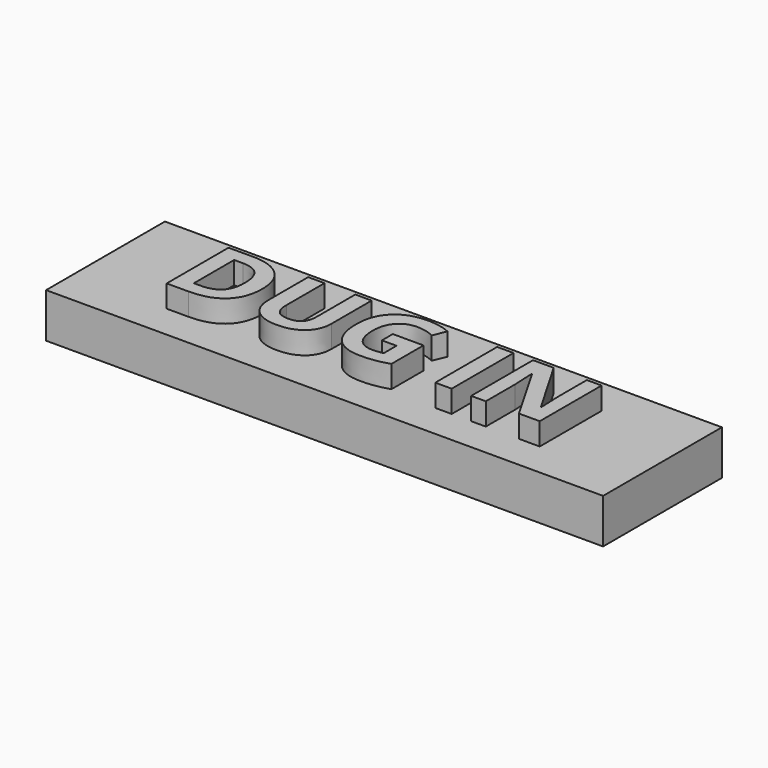
from build123d import *

# Parameters (mm, degrees)
F0_W         = 25
F0_H         = 6.6666666667
F1_DEPTH     = 2
F2_TEXT_SIZE = 4.8611111111
F3_DEPTH     = 1


# Not quite as in the source:
# - Text() gives the source's letters only with a copy of the font that has no kerning and outlines rounded to 1/6400 em; it was checked with that copy


with BuildPart() as f1:
    # F0 (on Top) → F1 (new body)
    with BuildSketch(Plane.XY):
        with Locations((-38.2137671113, 26.4245305329)):
            Rectangle(F0_W, F0_H)
    extrude(amount=F1_DEPTH)

    # F2 (on face) → F3 (join)
    with BuildSketch(Plane.XY.offset(2)):
        with Locations((-46.9680666145, 24.6287553559)):
            Text('DUG IN', F2_TEXT_SIZE, font='Open Sans', font_style=FontStyle.BOLD, text_align=(TextAlign.LEFT, TextAlign.BOTTOM))
    extrude(amount=F3_DEPTH)


solid = f1.part
